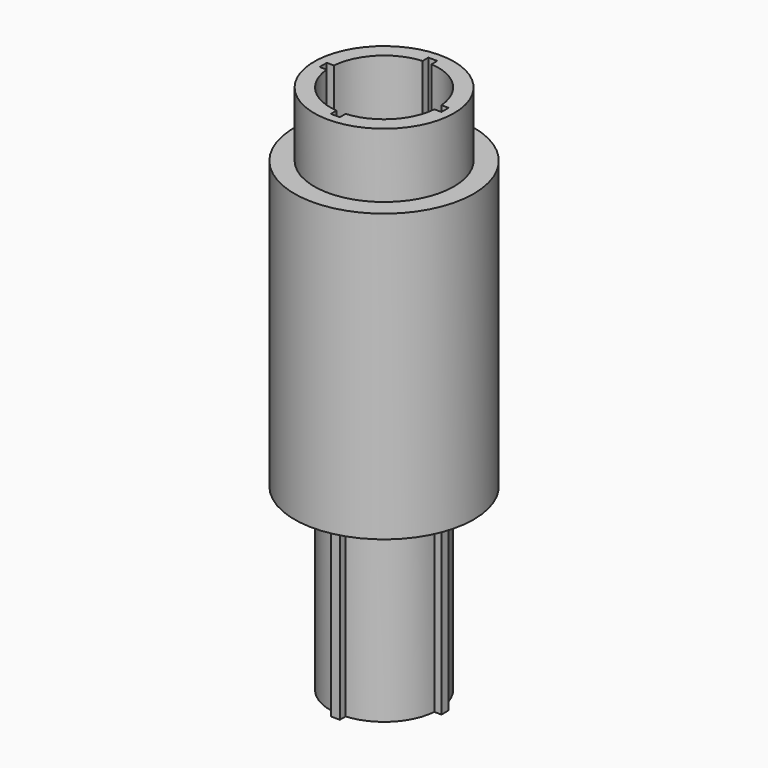
from build123d import *

# Parameters (mm, degrees)
F0_R     = 24.765
F1_DEPTH = 22.86
F2_R     = 31.75
F2_R_2   = 24.765
F3_DEPTH = 101.6
F6_DEPTH = 62.23
F7_DEPTH = 63.5


# Not quite as in the source:
# - a pattern or mirror of a feature is missing from the dataset's text; its kind, count and spacing are read off the source's solid


with BuildPart() as f1:
    # F0 (on Top) → F1 (new body)
    with BuildSketch(Plane.XY):
        Circle(F0_R)
    extrude(amount=F1_DEPTH)

    # F2 (on face) → F3 (join)
    with BuildSketch(Plane(origin=(0, 0, 0), x_dir=(1, 0, 0), z_dir=(0, 0, -1))):
        Circle(F2_R)
        Circle(F2_R_2, mode=Mode.SUBTRACT)
        Circle(F2_R_2)
    extrude(amount=F3_DEPTH)

    # F5 (on face) → F6 (cut)
    with BuildSketch(Plane.XY.offset(22.86)):
        with BuildLine():
            Line((-21.59, 1.5875), (-21.59, 0))
            Line((-21.59, 0), (-21.59, -1.5875))
            Line((-21.59, -1.5875), (-19.05, -1.5875))
            ThreePointArc((-19.05, -1.5875), (-13.517075428, -13.517075428), (-1.5875, -19.05))
            Line((-1.5875, -19.05), (-1.5875, -21.59))
            Line((-1.5875, -21.59), (1.5875, -21.59))
            Line((1.5875, -21.59), (1.5875, -19.05))
            ThreePointArc((1.5875, -19.05), (13.517075428, -13.517075428), (19.05, -1.5875))
            Line((19.05, -1.5875), (21.59, -1.5875))
            Line((21.59, -1.5875), (21.59, 0))
            Line((21.59, 0), (21.59, 1.5875))
            Line((21.59, 1.5875), (19.05, 1.5875))
            ThreePointArc((19.05, 1.5875), (13.517075428, 13.517075428), (1.5875, 19.05))
            Line((1.5875, 19.05), (1.5875, 21.59))
            Line((1.5875, 21.59), (-1.5875, 21.59))
            Line((-1.5875, 21.59), (-1.5875, 19.05))
            ThreePointArc((-1.5875, 19.05), (-13.517075428, 13.517075428), (-19.05, 1.5875))
            Line((-19.05, 1.5875), (-21.59, 1.5875))
        make_face()
    extrude(amount=-F6_DEPTH, mode=Mode.SUBTRACT)

    # F4 (on face) → F7 (join)
    with BuildSketch(Plane(origin=(0, 0, -101.6), x_dir=(1, 0, 0), z_dir=(0, 0, -1))):
        with BuildLine():
            Line((-21.59, 1.5875), (-21.59, 0))
            Line((-21.59, 0), (-21.59, -1.5875))
            Line((-21.59, -1.5875), (-19.05, -1.5875))
            ThreePointArc((-19.05, -1.5875), (-13.517075428, -13.517075428), (-1.5875, -19.05))
            Line((-1.5875, -19.05), (-1.5875, -21.59))
            Line((-1.5875, -21.59), (1.5875, -21.59))
            Line((1.5875, -21.59), (1.5875, -19.05))
            ThreePointArc((1.5875, -19.05), (13.517075428, -13.517075428), (19.05, -1.5875))
            Line((19.05, -1.5875), (21.59, -1.5875))
            Line((21.59, -1.5875), (21.59, 0))
            Line((21.59, 0), (21.59, 1.5875))
            Line((21.59, 1.5875), (19.05, 1.5875))
            ThreePointArc((19.05, 1.5875), (13.517075428, 13.517075428), (1.5875, 19.05))
            Line((1.5875, 19.05), (1.5875, 21.59))
            Line((1.5875, 21.59), (-1.5875, 21.59))
            Line((-1.5875, 21.59), (-1.5875, 19.05))
            ThreePointArc((-1.5875, 19.05), (-13.517075428, 13.517075428), (-19.05, 1.5875))
            Line((-19.05, 1.5875), (-21.59, 1.5875))
        make_face()
    f7 = extrude(amount=F7_DEPTH)

    # F7_copies: F7 across plane
    add(f7.mirror(Plane.XY.offset(-102.235)))


solid = f1.part
